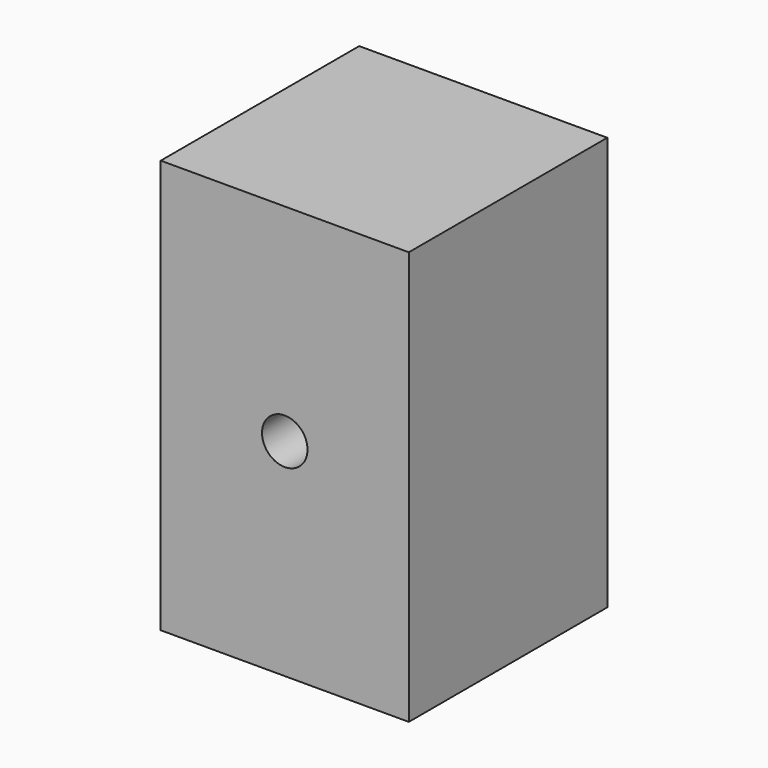
from build123d import *

# Parameters (mm, degrees)
F0_W     = 120
F0_H     = 200
F1_DEPTH = 120
F3_D     = 22


# Not quite as in the source:
# - a feature names something its author has since deleted; it is built from what else it names


with BuildPart() as f1:
    # F0 (on Front) → F1 (new body)
    with BuildSketch(Plane.XZ):
        Rectangle(F0_W, F0_H)
    extrude(amount=F1_DEPTH)

    # F3 (through all)
    with Locations(Plane.XZ.offset(120)):
        with Locations((0, 0)):
            Hole(F3_D / 2)


solid = f1.part
